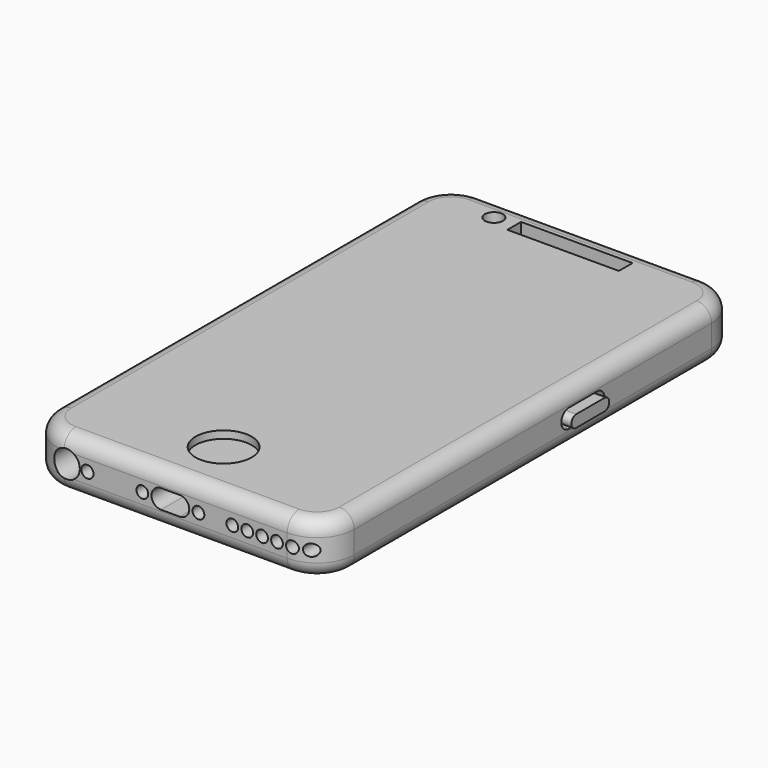
from build123d import *

# Parameters (mm, degrees)
F0_W          = 40
F0_H          = 70
F1_DEPTH      = 7
F2_R          = 0.7899610996
F2_R_2        = 0.7879667618
F2_R_3        = 1.8073925599
F2_R_4        = 0.8167266128
F3_DEPTH      = 10
F5_DEPTH      = 12
F7_DEPTH      = 13
F8_R          = 3.7758905803
F9_DEPTH      = 1
F10_W         = 14.9725805968
F10_H         = 2.3034736514
F10_R         = 1.22160092
F11_DEPTH     = 2
F12_T1_DEPTH  = 32
F13_R         = 5
F14_R         = 5
F15_T1_DEPTH  = 32
F16_T1_DEPTH  = 60
F16_T3_DEPTH  = 30
F16_T6_ANGLE  = 90
F16_T8_ANGLE  = 89.9999999974
F16_T10_ANGLE = 89.9999999974
F16_T12_ANGLE = 90
F17_T1_DEPTH  = 60
F17_T3_DEPTH  = 30
F17_T6_ANGLE  = 90
F17_T8_ANGLE  = 89.9999999974
F17_T10_ANGLE = 89.9999999974
F17_T12_ANGLE = 90


# Not quite as in the source:
# - a fillet or chamfer that OpenCascade refuses, or shapes differently, is made with other operations: its cross-section is extruded or revolved along the edge and cut away or added
# - ends of sketch curves that miss each other by under 0.0002 mm in the source are joined


with BuildPart() as f1:
    # F0 (on Top) → F1 (new body)
    with BuildSketch(Plane.XY):
        with Locations((20, 35)):
            Rectangle(F0_W, F0_H)
    extrude(amount=F1_DEPTH)

    # F2 (on face) → F3 (cut)
    with BuildSketch(Plane.XZ):
        with Locations((15.5336856842, 3.5)):
            Circle(F2_R)
        with BuildLine():
            Line((20.5575972795, 4.779751625), (18.0456396192, 4.779751625))
            ThreePointArc((18.0456396192, 4.779751625), (16.7658879943, 3.5), (18.0456396192, 2.220248375))
            Line((18.0456396192, 2.220248375), (20.5575972795, 2.220248375))
            ThreePointArc((20.5575972795, 2.220248375), (21.8373489045, 3.5), (20.5575972795, 4.779751625))
        make_face()
        with Locations((27.6224724948, 3.5)):
            Circle(F2_R_2)
        with Locations((23.0695530772, 3.5)):
            Circle(F2_R)
        with Locations((29.6224724948, 3.5)):
            Circle(F2_R_2)
        with Locations((31.6224724948, 3.5)):
            Circle(F2_R_2)
        with Locations((33.6224724948, 3.5)):
            Circle(F2_R_2)
        with Locations((35.6224724948, 3.5)):
            Circle(F2_R_2)
        with Locations((37.6224724948, 3.5)):
            Circle(F2_R_2)
        with Locations((5.3267837502, 3.5)):
            Circle(F2_R_3)
        with Locations((8.1548150629, 3.5)):
            Circle(F2_R_4)
    extrude(amount=-F3_DEPTH, mode=Mode.SUBTRACT)

    # F4 (on face) → F5 (cut)
    with BuildSketch(Plane.YZ.offset(40)):
        with BuildLine():
            Line((45.7730665803, 4.75), (41.0204045475, 4.75))
            ThreePointArc((41.0204045475, 4.75), (39.7704045475, 3.5000009306), (41.0204026863, 2.25))
            Line((41.0204026863, 2.25), (45.7730665803, 2.25))
            ThreePointArc((45.7730665803, 2.25), (47.0230665803, 3.5), (45.7730665803, 4.75))
        make_face()
    extrude(amount=-F5_DEPTH, mode=Mode.SUBTRACT)

    # F6 (on face) → F7 (join)
    with BuildSketch(Plane.YZ.offset(28)):
        with BuildLine():
            Line((45.7748817965, 4.3017610189), (41.022244125, 4.312521164))
            ThreePointArc((41.022244125, 4.312521164), (41.0213243392, 4.3125248082), (41.0204045475, 4.3125253288))
            ThreePointArc((41.0204045475, 4.3125253288), (40.2078792186, 3.5000009306), (41.0204026863, 2.6874746712))
            ThreePointArc((41.0204026863, 2.6874746712), (41.0213234086, 2.6874751907), (41.0222441297, 2.6874767536))
            Line((41.0222441297, 2.6874767536), (45.7748817965, 2.6982389853))
            ThreePointArc((45.7748817965, 2.6982389853), (46.5748296498, 3.5), (45.7748817965, 4.3017610189))
        make_face()
    extrude(amount=F7_DEPTH)

    # F8 (on face) → F9 (cut)
    with BuildSketch(Plane.XY.offset(7)):
        with Locations((20, 8.0621577799)):
            Circle(F8_R)
    extrude(amount=-F9_DEPTH, mode=Mode.SUBTRACT)

    # F10 (on face) → F11 (cut)
    with BuildSketch(Plane.XY.offset(7)):
        with Locations((19.9095932767, 66.3465745747)):
            Rectangle(F10_W, F10_H)
        with Locations((9.5746694133, 66.4882957935)):
            Circle(F10_R)
    extrude(amount=-F11_DEPTH, mode=Mode.SUBTRACT)

    # F12: fillet of radius 5 on 1 edges, made by hand

    # F12_s2 → F12_t1 (cut)
    with BuildSketch(Plane.XY.offset(-12.5)):
        with BuildLine():
            ThreePointArc((0, 5), (1.4644660941, 1.4644660941), (5, 0))
            Line((5, 0), (0, 0))
            Line((0, 0), (0, 5))
        make_face()
    extrude(amount=F12_T1_DEPTH, mode=Mode.SUBTRACT)

    # F13
    f13_edges = [f1.edges().sort_by_distance(p)[0] for p in [
        (0, 70, 3.5),
    ]]
    fillet(f13_edges, radius=F13_R)

    # F14
    f14_edges = [f1.edges().sort_by_distance(p)[0] for p in [
        (40, 70, 3.5),
    ]]
    fillet(f14_edges, radius=F14_R)

    # F15: fillet of radius 5 on 1 edges, made by hand

    # F15_s2 → F15_t1 (cut)
    with BuildSketch(Plane.XY.offset(-12.5)):
        with BuildLine():
            ThreePointArc((40, 5), (38.5355339059, 1.4644660941), (35, 0))
            Line((35, 0), (40, 0))
            Line((40, 0), (40, 5))
        make_face()
    extrude(amount=F15_T1_DEPTH, mode=Mode.SUBTRACT)

    # F16: fillet of radius 2 on 2 edges, made by hand

    # F16_s2 → F16_t1 (cut)
    with BuildSketch(Plane.XZ.offset(-65)):
        with BuildLine():
            ThreePointArc((40, 5), (39.4142135624, 6.4142135624), (38, 7))
            Line((38, 7), (40, 7))
            Line((40, 7), (40, 5))
        make_face()
        with BuildLine():
            ThreePointArc((0, 5), (0.5857864376, 6.4142135624), (2, 7))
            Line((2, 7), (0, 7))
            Line((0, 7), (0, 5))
        make_face()
    extrude(amount=F16_T1_DEPTH, mode=Mode.SUBTRACT)

    # F16_s4 → F16_t3 (cut)
    with BuildSketch(Plane.YZ.offset(5)):
        with BuildLine():
            ThreePointArc((0, 5), (0.5857864376, 6.4142135624), (2, 7))
            Line((2, 7), (0, 7))
            Line((0, 7), (0, 5))
        make_face()
        with BuildLine():
            ThreePointArc((70, 5), (69.4142135624, 6.4142135624), (68, 7))
            Line((68, 7), (70, 7))
            Line((70, 7), (70, 5))
        make_face()
    extrude(amount=F16_T3_DEPTH, mode=Mode.SUBTRACT)

    # F16_s5 → F16_t6 (revolve, cut)
    with BuildSketch(Plane.XZ.offset(-65)):
        with BuildLine():
            ThreePointArc((0, 5), (0.5857864376, 6.4142135624), (2, 7))
            Line((2, 7), (0, 7))
            Line((0, 7), (0, 5))
        make_face()
    revolve(axis=Axis((5, 65, 7), (0, 0, -1)), revolution_arc=F16_T6_ANGLE, mode=Mode.SUBTRACT)

    # F16_s7 → F16_t8 (revolve, cut)
    with BuildSketch(Plane.YZ.offset(5.0000000001)):
        with BuildLine():
            ThreePointArc((0, 5), (0.5857864376, 6.4142135624), (2, 7))
            Line((2, 7), (0, 7))
            Line((0, 7), (0, 5))
        make_face()
    revolve(axis=Axis((5.0000000001, 5.0000000001, 7), (0, 0, -1)), revolution_arc=F16_T8_ANGLE, mode=Mode.SUBTRACT)

    # F16_s9 → F16_t10 (revolve, cut)
    with BuildSketch(Plane.XZ.offset(-5.0000000001)):
        with BuildLine():
            ThreePointArc((40, 5), (39.4142135624, 6.4142135624), (38, 7))
            Line((38, 7), (40, 7))
            Line((40, 7), (40, 5))
        make_face()
    revolve(axis=Axis((34.9999999999, 5.0000000001, 7), (0, 0, -1)), revolution_arc=F16_T10_ANGLE, mode=Mode.SUBTRACT)

    # F16_s11 → F16_t12 (revolve, cut)
    with BuildSketch(Plane.YZ.offset(35)):
        with BuildLine():
            ThreePointArc((70, 5), (69.4142135624, 6.4142135624), (68, 7))
            Line((68, 7), (70, 7))
            Line((70, 7), (70, 5))
        make_face()
    revolve(axis=Axis((35, 65, 7), (0, 0, -1)), revolution_arc=F16_T12_ANGLE, mode=Mode.SUBTRACT)

    # F17: fillet of radius 2 on 8 edges, made by hand

    # F17_s2 → F17_t1 (cut)
    with BuildSketch(Plane.XZ.offset(-65)):
        with BuildLine():
            ThreePointArc((2, 0), (0.5857864376, 0.5857864376), (0, 2))
            Line((0, 2), (0, 0))
            Line((0, 0), (2, 0))
        make_face()
        with BuildLine():
            ThreePointArc((38, 0), (39.4142135624, 0.5857864376), (40, 2))
            Line((40, 2), (40, 0))
            Line((40, 0), (38, 0))
        make_face()
    extrude(amount=F17_T1_DEPTH, mode=Mode.SUBTRACT)

    # F17_s4 → F17_t3 (cut)
    with BuildSketch(Plane.YZ.offset(5)):
        with BuildLine():
            ThreePointArc((2, 0), (0.5857864376, 0.5857864376), (0, 2))
            Line((0, 2), (0, 0))
            Line((0, 0), (2, 0))
        make_face()
        with BuildLine():
            ThreePointArc((68, 0), (69.4142135624, 0.5857864376), (70, 2))
            Line((70, 2), (70, 0))
            Line((70, 0), (68, 0))
        make_face()
    extrude(amount=F17_T3_DEPTH, mode=Mode.SUBTRACT)

    # F17_s5 → F17_t6 (revolve, cut)
    with BuildSketch(Plane.YZ.offset(35)):
        with BuildLine():
            ThreePointArc((68, 0), (69.4142135624, 0.5857864376), (70, 2))
            Line((70, 2), (70, 0))
            Line((70, 0), (68, 0))
        make_face()
    revolve(axis=Axis((35, 65, 0), (0, 0, -1)), revolution_arc=F17_T6_ANGLE, mode=Mode.SUBTRACT)

    # F17_s7 → F17_t8 (revolve, cut)
    with BuildSketch(Plane.XZ.offset(-5.0000000001)):
        with BuildLine():
            ThreePointArc((38, 0), (39.4142135624, 0.5857864376), (40, 2))
            Line((40, 2), (40, 0))
            Line((40, 0), (38, 0))
        make_face()
    revolve(axis=Axis((34.9999999999, 5.0000000001, 0), (0, 0, -1)), revolution_arc=F17_T8_ANGLE, mode=Mode.SUBTRACT)

    # F17_s9 → F17_t10 (revolve, cut)
    with BuildSketch(Plane.YZ.offset(5.0000000001)):
        with BuildLine():
            ThreePointArc((2, 0), (0.5857864376, 0.5857864376), (0, 2))
            Line((0, 2), (0, 0))
            Line((0, 0), (2, 0))
        make_face()
    revolve(axis=Axis((5.0000000001, 5.0000000001, 0), (0, 0, -1)), revolution_arc=F17_T10_ANGLE, mode=Mode.SUBTRACT)

    # F17_s11 → F17_t12 (revolve, cut)
    with BuildSketch(Plane.XZ.offset(-65)):
        with BuildLine():
            ThreePointArc((2, 0), (0.5857864376, 0.5857864376), (0, 2))
            Line((0, 2), (0, 0))
            Line((0, 0), (2, 0))
        make_face()
    revolve(axis=Axis((5, 65, 0), (0, 0, -1)), revolution_arc=F17_T12_ANGLE, mode=Mode.SUBTRACT)


solid = f1.part
